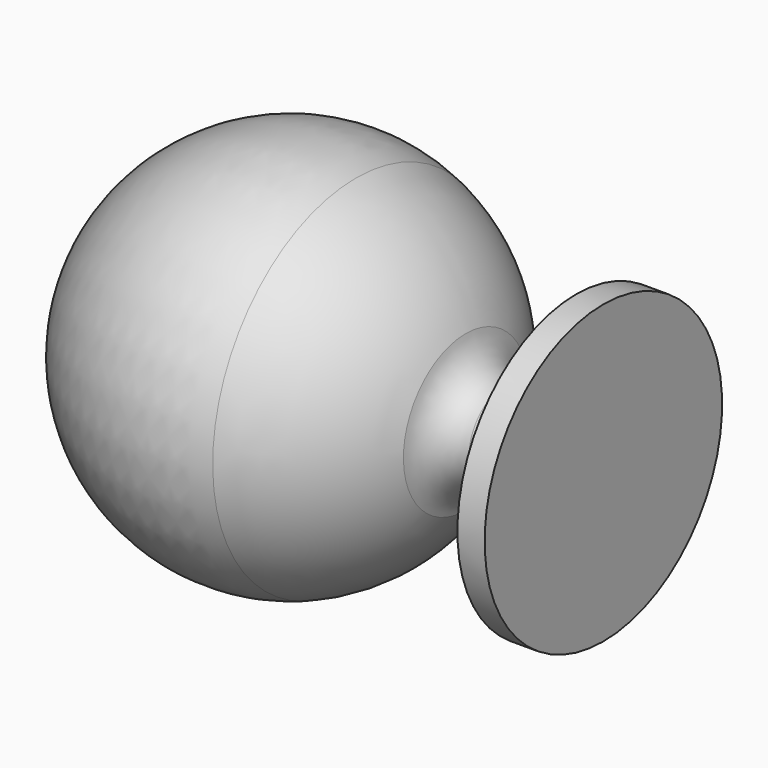
from build123d import *


# Not quite as in the source:
# - a fillet or chamfer that OpenCascade refuses, or shapes differently, is made with other operations: its cross-section is extruded or revolved along the edge and cut away or added


with BuildPart() as f1:
    # F0 (on Front) → F1 (revolve)
    with BuildSketch(Plane.XZ):
        with BuildLine():
            ThreePointArc((46.5161651373, 9.8678171635), (40.8437195411, 17.6691792738), (32.6236449182, 22.7157883346))
            ThreePointArc((32.6236449182, 22.7157883346), (10.4441791353, 19.7848045383), (0, 0))
            Line((0, 0), (60.5131424963, 0))
            Line((60.5131424963, 0), (63.9651343226, 0))
            Line((63.9651343226, 0), (63.9651343226, 18.8124477863))
            Line((63.9651343226, 18.8124477863), (60.5131424963, 18.8124477863))
            Line((60.5131424963, 18.8124477863), (60.5131424963, 11.1212786287))
            Line((60.5131424963, 11.1212786287), (60.5131424963, 5.7427594438))
            Line((60.5131424963, 5.7427594438), (46.5161651373, 5.7427594438))
            Line((46.5161651373, 5.7427594438), (46.5161651373, 9.8678171635))
        make_face()
    revolve(axis=Axis((30.2565712482, 0, 0), (1, 0, 0)))

    # F2: fillet of radius 5.08 on 2 edges, made by hand

    # F2_s1 → F2_t2 (revolve)
    with BuildSketch(Plane.XZ):
        with BuildLine():
            ThreePointArc((51.5056025045, 5.7427594438), (48.2686831963, 6.9075642517), (46.5161651373, 9.8678171635))
            Line((46.5161651373, 9.8678171635), (46.4163763899, 9.8487183179))
            ThreePointArc((46.4163763899, 9.8487183179), (46.4145651373, 7.8052883036), (46.4145651373, 5.7427594438))
            Line((46.4145651373, 5.7427594438), (46.5161651373, 5.6411594438))
            Line((46.5161651373, 5.6411594438), (51.5056025045, 5.6411594438))
            Line((51.5056025045, 5.6411594438), (51.5056025045, 5.7427594438))
        make_face()
    revolve(axis=Axis((46.5161651373, 0, 0), (1, 0, 0)))

    # F2_s3 → F2_t4 (revolve)
    with BuildSketch(Plane.XZ):
        with BuildLine():
            ThreePointArc((60.5131424963, 10.8227594438), (59.0252449448, 7.2306569954), (55.4331424963, 5.7427594438))
            Line((55.4331424963, 5.7427594438), (55.4331424963, 5.6411594438))
            Line((55.4331424963, 5.6411594438), (60.6147424963, 5.6411594438))
            Line((60.6147424963, 5.6411594438), (60.6147424963, 10.8227594438))
            Line((60.6147424963, 10.8227594438), (60.5131424963, 10.8227594438))
        make_face()
    revolve(axis=Axis((60.5131424963, 0, 0), (1, 0, 0)))


solid = f1.part
